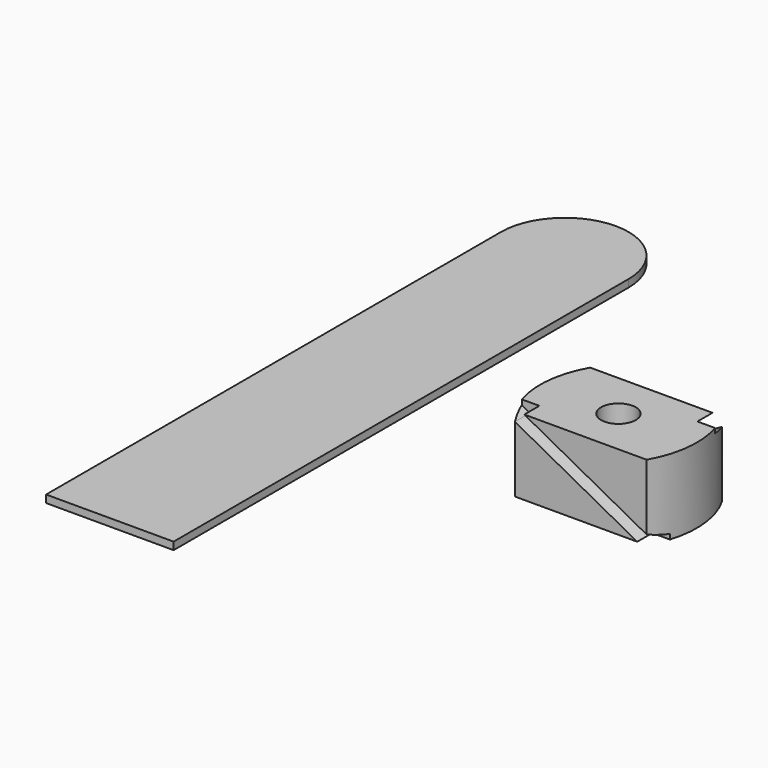
from build123d import *

# Parameters (mm, degrees)
F1_DEPTH = 10.16
F3_DEPTH = 2.54
F5_DEPTH = 2.54
F6_R     = 2.341346142
F7_DEPTH = 10.161
F9_DEPTH = 1.016


# Not quite as in the source:
# - a feature names something its author has since deleted; it is built from what else it names


with BuildPart() as f1:
    # F0 (on Top) → F1 (new body)
    with BuildSketch(Plane.XY):
        with BuildLine():
            ThreePointArc((-8.89, 6.35), (-10.5782148046, 0), (-8.89, -6.35))
            Line((-8.89, -6.35), (0, -6.35))
            Line((0, -6.35), (0, 6.35))
            Line((0, 6.35), (-8.89, 6.35))
        make_face()
        with BuildLine():
            Line((0, 6.35), (0, -6.35))
            Line((0, -6.35), (8.89, -6.35))
            ThreePointArc((8.89, -6.35), (10.5782148046, 0), (8.89, 6.35))
            Line((8.89, 6.35), (0, 6.35))
        make_face()
    extrude(amount=F1_DEPTH)

    # F2 (on face) → F3 (cut)
    with BuildSketch(Plane.XZ.offset(6.35)):
        Polygon((11.2485714286, 0), (8.89, 1.27), (-7.62, 10.16), (-8.89, 10.16), (-11.2485714286, 10.16), (-8.89, 8.89), (7.62, 0), (8.89, 0), align=None)
    extrude(amount=-F3_DEPTH, mode=Mode.SUBTRACT)

    # F4 (on face) → F5 (cut)
    with BuildSketch(Plane(origin=(0, 6.35, 0), x_dir=(-1, 0, 0), z_dir=(0, 1, 0))):
        Polygon((8.89, 1.27), (0, 6.0569230769), (0, 4.1030769231), (7.62, 0), (11.2485714286, 0), align=None)
        Polygon((0, 4.1030769231), (0, 6.0569230769), (-7.62, 10.16), (-11.2485714286, 10.16), (-8.89, 8.89), align=None)
    extrude(amount=-F5_DEPTH, mode=Mode.SUBTRACT)

    # F6 (on face) → F7 (cut, through all)
    with BuildSketch(Plane.XY.offset(10.16)):
        Circle(F6_R)
    extrude(amount=-F7_DEPTH, mode=Mode.SUBTRACT)


with BuildPart() as f9:
    # F8 (on Top) → F9 (new body)
    with BuildSketch(Plane.XY):
        with BuildLine():
            Line((-46.5480796993, 38.3802093565), (-46.5480796993, -38.3802093565))
            Line((-46.5480796993, -38.3802093565), (-29.3340720236, -38.3802093565))
            Line((-29.3340720236, -38.3802093565), (-29.3340720236, 38.3802093565))
            ThreePointArc((-29.3340720236, 38.3802093565), (-37.9410758615, 46.9872131944), (-46.5480796993, 38.3802093565))
        make_face()
    extrude(amount=F9_DEPTH)


solid = Compound([f1.part, f9.part])
